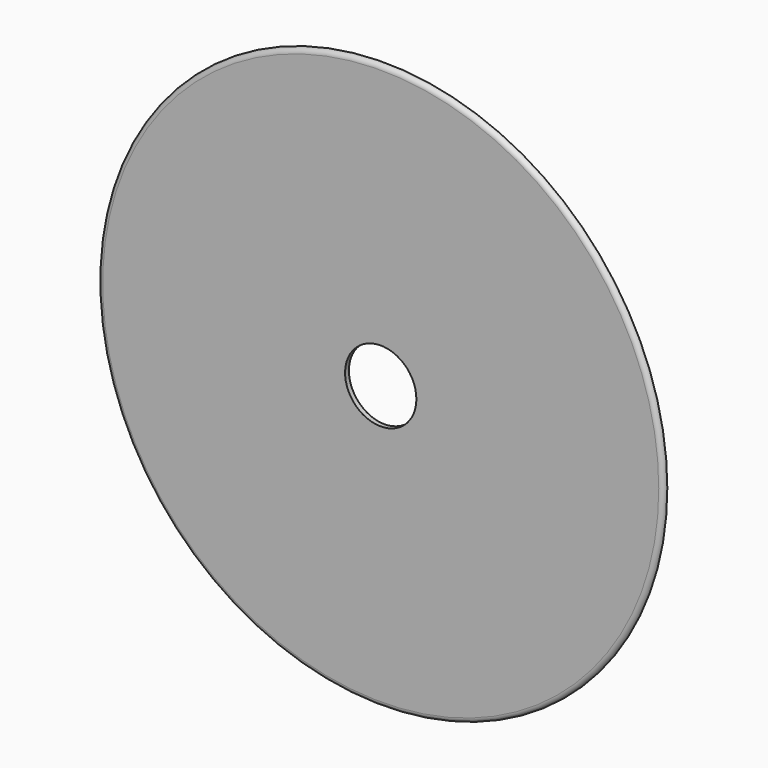
from build123d import *

# Parameters (mm, degrees)
F0_R     = 59.5
F0_R_2   = 7.5
F1_DEPTH = 1
F2_R     = 0.99999


# Not quite as in the source:
# - a fillet or chamfer is up to 0.001 mm smaller than in the source, because OpenCascade refuses the exact size


with BuildPart() as f1:
    # F0 (on Front) → F1 (new body)
    with BuildSketch(Plane.XZ):
        Circle(F0_R)
        Circle(F0_R_2, mode=Mode.SUBTRACT)
    extrude(amount=F1_DEPTH)

    # F2 (radius 1 in the source; OpenCascade refuses exactly that, so slightly less here)
    f2_edges = [f1.edges().sort_by_distance(p)[0] for p in [
        (-59.5, -1, 0),
    ]]
    fillet(f2_edges, radius=F2_R)


solid = f1.part
